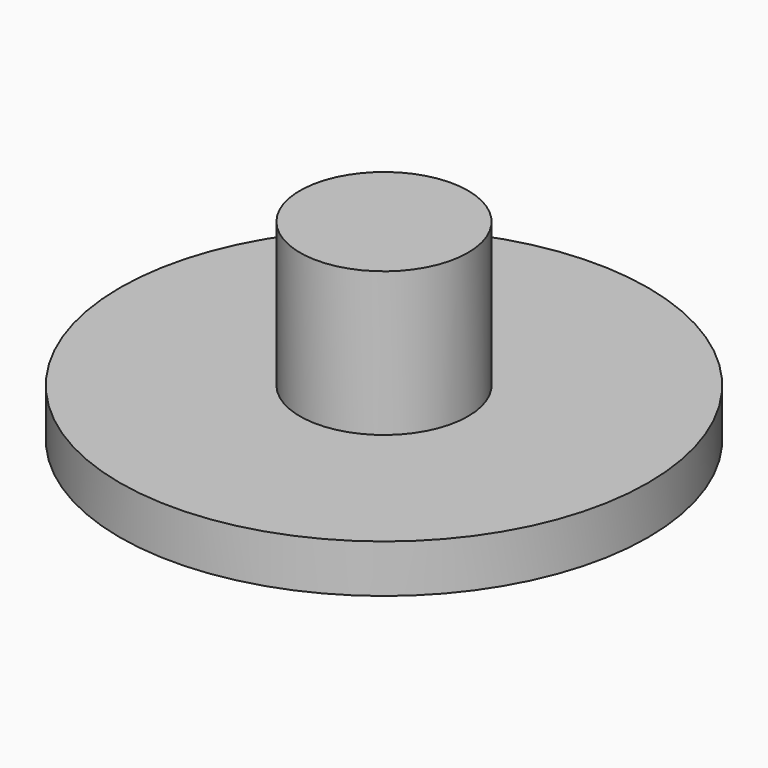
from build123d import *

# Parameters (mm, degrees)
F0_R     = 3.5
F1_DEPTH = 6
F2_R     = 11
F2_R_2   = 3.5
F3_DEPTH = 2


with BuildPart() as f1:
    # F0 (on Top) → F1 (new body)
    with BuildSketch(Plane.XY):
        Circle(F0_R)
    extrude(amount=F1_DEPTH)

    # F2 (on face) → F3 (join)
    with BuildSketch(Plane(origin=(0, 0, 0), x_dir=(1, 0, 0), z_dir=(0, 0, -1))):
        Circle(F2_R)
        Circle(F2_R_2, mode=Mode.SUBTRACT)
        Circle(F2_R_2)
    extrude(amount=F3_DEPTH)


solid = f1.part
